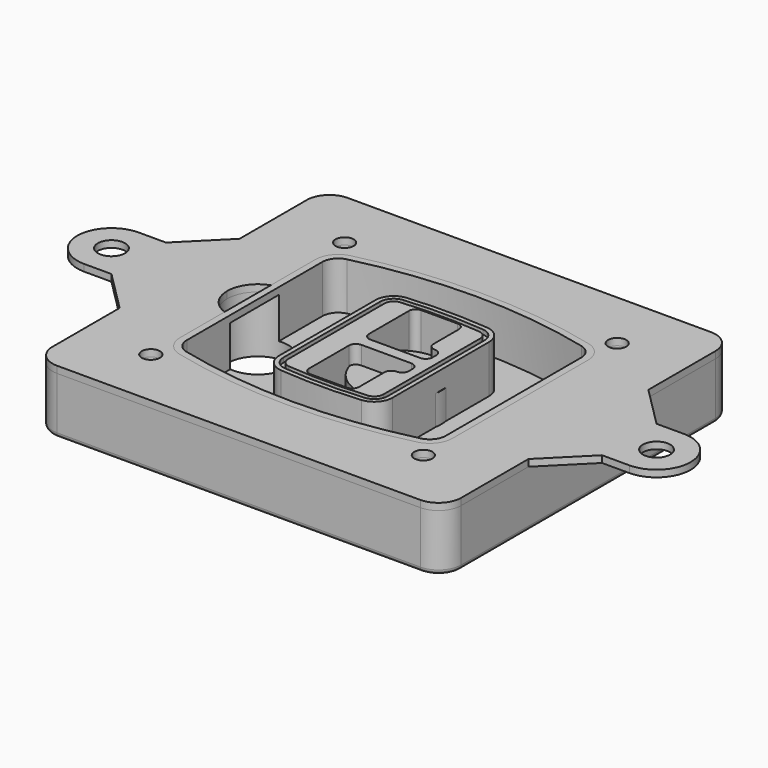
from build123d import *

# Parameters (mm, degrees)
F0_R      = 4
F1_DEPTH  = 25
F2_DEPTH  = 3
F3_DEPTH  = 18
F5_DEPTH  = 21
F6_DEPTH  = 2
F8_DEPTH  = 20
F9_DEPTH  = 16
F10_DEPTH = 25
F7_R      = 6
F7_R_2    = 4
F11_DEPTH = 6
F13_DEPTH = 9
F15_R     = 2
F16_R     = 4
F16_R_2   = 6
F17_DEPTH = 3


# Not quite as in the source:
# - a feature of the source that left no trace in its solid (it failed there, or was rolled back) is left out
# - a feature names something its author has since deleted; it is built from what else it names


with BuildPart() as f1:
    # F0 (on Top) → F1 (new body)
    with BuildSketch(Plane.XY):
        with BuildLine():
            ThreePointArc((-90, -70), (-87.0710678119, -77.0710678119), (-80, -80))
            Line((-80, -80), (80, -80))
            ThreePointArc((80, -80), (87.0710678119, -77.0710678119), (90, -70))
            Line((90, -70), (90, 70))
            ThreePointArc((90, 70), (87.0710678119, 77.0710678119), (80, 80))
            Line((80, 80), (-80, 80))
            ThreePointArc((-80, 80), (-87.0710678119, 77.0710678119), (-90, 70))
            Line((-90, 70), (-90, -70))
        make_face()
        with Locations((-60, -53.3333333333)):
            Circle(F0_R, mode=Mode.SUBTRACT)
        with Locations((60, -53.3333333333)):
            Circle(F0_R, mode=Mode.SUBTRACT)
        with Locations((-60, 53.3333333333)):
            Circle(F0_R, mode=Mode.SUBTRACT)
        with BuildLine():
            ThreePointArc((-64, 37.2990447398), (-61.0143011354, 45.9411029726), (-53.3306899286, 50.8970778549))
            ThreePointArc((-53.3306899286, 50.8970778549), (0, 57.3333333333), (53.3306899286, 50.8970778549))
            ThreePointArc((53.3306899286, 50.8970778549), (61.0143011354, 45.9411029726), (64, 37.2990447398))
            Line((64, 37.2990447398), (64, -37.2990447398))
            ThreePointArc((64, -37.2990447398), (61.0143011354, -45.9411029726), (53.3306899286, -50.8970778549))
            ThreePointArc((53.3306899286, -50.8970778549), (0, -57.3333333333), (-53.3306899286, -50.8970778549))
            ThreePointArc((-53.3306899286, -50.8970778549), (-61.0143011354, -45.9411029726), (-64, -37.2990447398))
            Line((-64, -37.2990447398), (-64, 37.2990447398))
        make_face(mode=Mode.SUBTRACT)
        with Locations((60, 53.3333333333)):
            Circle(F0_R, mode=Mode.SUBTRACT)
        with BuildLine():
            ThreePointArc((53.3306899286, 50.8970778549), (0, 57.3333333333), (-53.3306899286, 50.8970778549))
            ThreePointArc((-53.3306899286, 50.8970778549), (-61.0143011354, 45.9411029726), (-64, 37.2990447398))
            Line((-64, 37.2990447398), (-64, -37.2990447398))
            ThreePointArc((-64, -37.2990447398), (-61.0143011354, -45.9411029726), (-53.3306899286, -50.8970778549))
            ThreePointArc((-53.3306899286, -50.8970778549), (0, -57.3333333333), (53.3306899286, -50.8970778549))
            ThreePointArc((53.3306899286, -50.8970778549), (61.0143011354, -45.9411029726), (64, -37.2990447398))
            Line((64, -37.2990447398), (64, 37.2990447398))
            ThreePointArc((64, 37.2990447398), (61.0143011354, 45.9411029726), (53.3306899286, 50.8970778549))
        make_face()
        with BuildLine():
            Line((-60, -37.2990447398), (-60, 37.2990447398))
            ThreePointArc((-60, 37.2990447398), (-57.8673579538, 43.4719434775), (-52.3790642347, 47.0119255363))
            ThreePointArc((-52.3790642347, 47.0119255363), (0, 53.3333333333), (52.3790642347, 47.0119255363))
            ThreePointArc((52.3790642347, 47.0119255363), (57.8673579538, 43.4719434775), (60, 37.2990447398))
            Line((60, 37.2990447398), (60, -37.2990447398))
            ThreePointArc((60, -37.2990447398), (57.8673579538, -43.4719434775), (52.3790642347, -47.0119255363))
            ThreePointArc((52.3790642347, -47.0119255363), (0, -53.3333333333), (-52.3790642347, -47.0119255363))
            ThreePointArc((-52.3790642347, -47.0119255363), (-57.8673579538, -43.4719434775), (-60, -37.2990447398))
        make_face(mode=Mode.SUBTRACT)
        with BuildLine():
            ThreePointArc((-52.3790642347, 47.0119255363), (-57.8673579538, 43.4719434775), (-60, 37.2990447398))
            Line((-60, 37.2990447398), (-60, -37.2990447398))
            ThreePointArc((-60, -37.2990447398), (-57.8673579538, -43.4719434775), (-52.3790642347, -47.0119255363))
            ThreePointArc((-52.3790642347, -47.0119255363), (0, -53.3333333333), (52.3790642347, -47.0119255363))
            ThreePointArc((52.3790642347, -47.0119255363), (57.8673579538, -43.4719434775), (60, -37.2990447398))
            Line((60, -37.2990447398), (60, 37.2990447398))
            ThreePointArc((60, 37.2990447398), (57.8673579538, 43.4719434775), (52.3790642347, 47.0119255363))
            ThreePointArc((52.3790642347, 47.0119255363), (0, 53.3333333333), (-52.3790642347, 47.0119255363))
        make_face()
        with BuildLine():
            ThreePointArc((51.6653449643, 44.0980612973), (55.5071505677, 41.6200738562), (57, 37.2990447398))
            Line((57, 37.2990447398), (57, -37.2990447398))
            ThreePointArc((57, -37.2990447398), (55.5071505677, -41.6200738562), (51.6653449643, -44.0980612973))
            ThreePointArc((51.6653449643, -44.0980612973), (0, -50.3333333333), (-51.6653449643, -44.0980612973))
            ThreePointArc((-51.6653449643, -44.0980612973), (-55.5071505677, -41.6200738562), (-57, -37.2990447398))
            Line((-57, -37.2990447398), (-57, 37.2990447398))
            ThreePointArc((-57, 37.2990447398), (-55.5071505677, 41.6200738562), (-51.6653449643, 44.0980612973))
            ThreePointArc((-51.6653449643, 44.0980612973), (0, 50.3333333333), (51.6653449643, 44.0980612973))
        make_face(mode=Mode.SUBTRACT)
        with BuildLine():
            Line((57, -37.2990447398), (57, 37.2990447398))
            ThreePointArc((57, 37.2990447398), (55.5071505677, 41.6200738562), (51.6653449643, 44.0980612973))
            ThreePointArc((51.6653449643, 44.0980612973), (0, 50.3333333333), (-51.6653449643, 44.0980612973))
            ThreePointArc((-51.6653449643, 44.0980612973), (-55.5071505677, 41.6200738562), (-57, 37.2990447398))
            Line((-57, 37.2990447398), (-57, -37.2990447398))
            ThreePointArc((-57, -37.2990447398), (-55.5071505677, -41.6200738562), (-51.6653449643, -44.0980612973))
            ThreePointArc((-51.6653449643, -44.0980612973), (0, -50.3333333333), (51.6653449643, -44.0980612973))
            ThreePointArc((51.6653449643, -44.0980612973), (55.5071505677, -41.6200738562), (57, -37.2990447398))
        make_face()
    extrude(amount=-F1_DEPTH)

    # F0 (on Top) → F2 (join)
    with BuildSketch(Plane.XY):
        with BuildLine():
            ThreePointArc((-52.3790642347, 47.0119255363), (-57.8673579538, 43.4719434775), (-60, 37.2990447398))
            Line((-60, 37.2990447398), (-60, -37.2990447398))
            ThreePointArc((-60, -37.2990447398), (-57.8673579538, -43.4719434775), (-52.3790642347, -47.0119255363))
            ThreePointArc((-52.3790642347, -47.0119255363), (0, -53.3333333333), (52.3790642347, -47.0119255363))
            ThreePointArc((52.3790642347, -47.0119255363), (57.8673579538, -43.4719434775), (60, -37.2990447398))
            Line((60, -37.2990447398), (60, 37.2990447398))
            ThreePointArc((60, 37.2990447398), (57.8673579538, 43.4719434775), (52.3790642347, 47.0119255363))
            ThreePointArc((52.3790642347, 47.0119255363), (0, 53.3333333333), (-52.3790642347, 47.0119255363))
        make_face()
        with BuildLine():
            ThreePointArc((51.6653449643, 44.0980612973), (55.5071505677, 41.6200738562), (57, 37.2990447398))
            Line((57, 37.2990447398), (57, -37.2990447398))
            ThreePointArc((57, -37.2990447398), (55.5071505677, -41.6200738562), (51.6653449643, -44.0980612973))
            ThreePointArc((51.6653449643, -44.0980612973), (0, -50.3333333333), (-51.6653449643, -44.0980612973))
            ThreePointArc((-51.6653449643, -44.0980612973), (-55.5071505677, -41.6200738562), (-57, -37.2990447398))
            Line((-57, -37.2990447398), (-57, 37.2990447398))
            ThreePointArc((-57, 37.2990447398), (-55.5071505677, 41.6200738562), (-51.6653449643, 44.0980612973))
            ThreePointArc((-51.6653449643, 44.0980612973), (0, 50.3333333333), (51.6653449643, 44.0980612973))
        make_face(mode=Mode.SUBTRACT)
    extrude(amount=F2_DEPTH)

    # F0 (on Top) → F3 (cut)
    with BuildSketch(Plane.XY):
        with BuildLine():
            Line((57, -37.2990447398), (57, 37.2990447398))
            ThreePointArc((57, 37.2990447398), (55.5071505677, 41.6200738562), (51.6653449643, 44.0980612973))
            ThreePointArc((51.6653449643, 44.0980612973), (0, 50.3333333333), (-51.6653449643, 44.0980612973))
            ThreePointArc((-51.6653449643, 44.0980612973), (-55.5071505677, 41.6200738562), (-57, 37.2990447398))
            Line((-57, 37.2990447398), (-57, -37.2990447398))
            ThreePointArc((-57, -37.2990447398), (-55.5071505677, -41.6200738562), (-51.6653449643, -44.0980612973))
            ThreePointArc((-51.6653449643, -44.0980612973), (0, -50.3333333333), (51.6653449643, -44.0980612973))
            ThreePointArc((51.6653449643, -44.0980612973), (55.5071505677, -41.6200738562), (57, -37.2990447398))
        make_face()
    extrude(amount=-F3_DEPTH, mode=Mode.SUBTRACT)

    # F4 (on face) → F5 (join, through all)
    with BuildSketch(Plane.XY.offset(3)):
        with BuildLine():
            ThreePointArc((-25, -26.587695628), (-22.8992979869, -31.9912392117), (-17.7004291845, -34.5569740744))
            ThreePointArc((-17.7004291845, -34.5569740744), (0, -35.3333333333), (17.7004291845, -34.5569740744))
            ThreePointArc((17.7004291845, -34.5569740744), (22.8992979869, -31.9912392117), (25, -26.587695628))
            Line((25, -26.587695628), (25, 26.587695628))
            ThreePointArc((25, 26.587695628), (22.8992979869, 31.9912392117), (17.7004291845, 34.5569740744))
            ThreePointArc((17.7004291845, 34.5569740744), (0, 35.3333333333), (-17.7004291845, 34.5569740744))
            ThreePointArc((-17.7004291845, 34.5569740744), (-22.8992979869, 31.9912392117), (-25, 26.587695628))
            Line((-25, 26.587695628), (-25, -26.587695628))
        make_face()
        with BuildLine():
            ThreePointArc((17.5253218884, 32.5646544628), (21.4244734902, 30.6403533158), (23, 26.587695628))
            Line((23, 26.587695628), (23, -26.587695628))
            ThreePointArc((23, -26.587695628), (21.4244734902, -30.6403533158), (17.5253218884, -32.5646544628))
            ThreePointArc((17.5253218884, -32.5646544628), (0, -33.3333333333), (-17.5253218884, -32.5646544628))
            ThreePointArc((-17.5253218884, -32.5646544628), (-21.4244734902, -30.6403533158), (-23, -26.587695628))
            Line((-23, -26.587695628), (-23, 26.587695628))
            ThreePointArc((-23, 26.587695628), (-21.4244734902, 30.6403533158), (-17.5253218884, 32.5646544628))
            ThreePointArc((-17.5253218884, 32.5646544628), (0, 33.3333333333), (17.5253218884, 32.5646544628))
        make_face(mode=Mode.SUBTRACT)
        with BuildLine():
            Line((23, -26.587695628), (23, 26.587695628))
            ThreePointArc((23, 26.587695628), (21.4244734902, 30.6403533158), (17.5253218884, 32.5646544628))
            ThreePointArc((17.5253218884, 32.5646544628), (0, 33.3333333333), (-17.5253218884, 32.5646544628))
            ThreePointArc((-17.5253218884, 32.5646544628), (-21.4244734902, 30.6403533158), (-23, 26.587695628))
            Line((-23, 26.587695628), (-23, -26.587695628))
            ThreePointArc((-23, -26.587695628), (-21.4244734902, -30.6403533158), (-17.5253218884, -32.5646544628))
            ThreePointArc((-17.5253218884, -32.5646544628), (0, -33.3333333333), (17.5253218884, -32.5646544628))
            ThreePointArc((17.5253218884, -32.5646544628), (21.4244734902, -30.6403533158), (23, -26.587695628))
        make_face()
        with BuildLine():
            ThreePointArc((17.3502145923, 30.5723348512), (19.9496489934, 29.2894674198), (21, 26.587695628))
            Line((21, 26.587695628), (21, -26.587695628))
            ThreePointArc((21, -26.587695628), (19.9496489934, -29.2894674198), (17.3502145923, -30.5723348512))
            ThreePointArc((17.3502145923, -30.5723348512), (0, -31.3333333333), (-17.3502145923, -30.5723348512))
            ThreePointArc((-17.3502145923, -30.5723348512), (-19.9496489934, -29.2894674198), (-21, -26.587695628))
            Line((-21, -26.587695628), (-21, 26.587695628))
            ThreePointArc((-21, 26.587695628), (-19.9496489934, 29.2894674198), (-17.3502145923, 30.5723348512))
            ThreePointArc((-17.3502145923, 30.5723348512), (0, 31.3333333333), (17.3502145923, 30.5723348512))
        make_face(mode=Mode.SUBTRACT)
        with BuildLine():
            Line((21, -26.587695628), (21, 26.587695628))
            ThreePointArc((21, 26.587695628), (19.9496489934, 29.2894674198), (17.3502145923, 30.5723348512))
            ThreePointArc((17.3502145923, 30.5723348512), (0, 31.3333333333), (-17.3502145923, 30.5723348512))
            ThreePointArc((-17.3502145923, 30.5723348512), (-19.9496489934, 29.2894674198), (-21, 26.587695628))
            Line((-21, 26.587695628), (-21, -26.587695628))
            ThreePointArc((-21, -26.587695628), (-19.9496489934, -29.2894674198), (-17.3502145923, -30.5723348512))
            ThreePointArc((-17.3502145923, -30.5723348512), (0, -31.3333333333), (17.3502145923, -30.5723348512))
            ThreePointArc((17.3502145923, -30.5723348512), (19.9496489934, -29.2894674198), (21, -26.587695628))
        make_face()
        with BuildLine():
            Line((-8, -2.5), (14, -2.5))
            ThreePointArc((14, -2.5), (16.1213203436, -3.3786796564), (17, -5.5))
            Line((17, -5.5), (17, -7.5))
            ThreePointArc((17, -7.5), (16.1213203436, -9.6213203436), (14, -10.5))
            ThreePointArc((14, -10.5), (11.8786796564, -11.3786796564), (11, -13.5))
            Line((11, -13.5), (11, -27.5))
            ThreePointArc((11, -27.5), (10.1213203436, -29.6213203436), (8, -30.5))
            Line((8, -30.5), (-8, -30.5))
            ThreePointArc((-8, -30.5), (-10.1213203436, -29.6213203436), (-11, -27.5))
            Line((-11, -27.5), (-11, -5.5))
            ThreePointArc((-11, -5.5), (-10.1213203436, -3.3786796564), (-8, -2.5))
        make_face(mode=Mode.SUBTRACT)
        with BuildLine():
            ThreePointArc((-8, 2.5), (-10.1213203436, 3.3786796564), (-11, 5.5))
            Line((-11, 5.5), (-11, 27.5))
            ThreePointArc((-11, 27.5), (-10.1213203436, 29.6213203436), (-8, 30.5))
            Line((-8, 30.5), (8, 30.5))
            ThreePointArc((8, 30.5), (10.1213203436, 29.6213203436), (11, 27.5))
            Line((11, 27.5), (11, 13.5))
            ThreePointArc((11, 13.5), (11.8786796564, 11.3786796564), (14, 10.5))
            ThreePointArc((14, 10.5), (16.1213203436, 9.6213203436), (17, 7.5))
            Line((17, 7.5), (17, 5.5))
            ThreePointArc((17, 5.5), (16.1213203436, 3.3786796564), (14, 2.5))
            Line((14, 2.5), (-8, 2.5))
        make_face(mode=Mode.SUBTRACT)
    extrude(amount=-F5_DEPTH)

    # F4 (on face) → F6 (cut)
    with BuildSketch(Plane.XY.offset(3)):
        with BuildLine():
            Line((23, -26.587695628), (23, 26.587695628))
            ThreePointArc((23, 26.587695628), (21.4244734902, 30.6403533158), (17.5253218884, 32.5646544628))
            ThreePointArc((17.5253218884, 32.5646544628), (0, 33.3333333333), (-17.5253218884, 32.5646544628))
            ThreePointArc((-17.5253218884, 32.5646544628), (-21.4244734902, 30.6403533158), (-23, 26.587695628))
            Line((-23, 26.587695628), (-23, -26.587695628))
            ThreePointArc((-23, -26.587695628), (-21.4244734902, -30.6403533158), (-17.5253218884, -32.5646544628))
            ThreePointArc((-17.5253218884, -32.5646544628), (0, -33.3333333333), (17.5253218884, -32.5646544628))
            ThreePointArc((17.5253218884, -32.5646544628), (21.4244734902, -30.6403533158), (23, -26.587695628))
        make_face()
        with BuildLine():
            ThreePointArc((17.3502145923, 30.5723348512), (19.9496489934, 29.2894674198), (21, 26.587695628))
            Line((21, 26.587695628), (21, -26.587695628))
            ThreePointArc((21, -26.587695628), (19.9496489934, -29.2894674198), (17.3502145923, -30.5723348512))
            ThreePointArc((17.3502145923, -30.5723348512), (0, -31.3333333333), (-17.3502145923, -30.5723348512))
            ThreePointArc((-17.3502145923, -30.5723348512), (-19.9496489934, -29.2894674198), (-21, -26.587695628))
            Line((-21, -26.587695628), (-21, 26.587695628))
            ThreePointArc((-21, 26.587695628), (-19.9496489934, 29.2894674198), (-17.3502145923, 30.5723348512))
            ThreePointArc((-17.3502145923, 30.5723348512), (0, 31.3333333333), (17.3502145923, 30.5723348512))
        make_face(mode=Mode.SUBTRACT)
    extrude(amount=-F6_DEPTH, mode=Mode.SUBTRACT)

    # F7 (on face) → F8 (join)
    with BuildSketch(Plane(origin=(0, 0, -25), x_dir=(1, 0, 0), z_dir=(0, 0, -1))):
        with BuildLine():
            ThreePointArc((-6.71157564, 0), (6.7567035675, 13.4682792075), (20.224982775, 0))
            Line((20.224982775, 0), (25.224982775, 0))
            ThreePointArc((25.224982775, 0), (6.7567035675, 18.4682792075), (-11.71157564, 0))
            Line((-11.71157564, 0), (-6.71157564, 0))
        make_face()
        with BuildLine():
            Line((-6.71157564, 0), (20.224982775, 0))
            ThreePointArc((20.224982775, 0), (6.7567035675, 13.4682792075), (-6.71157564, 0))
        make_face()
        with BuildLine():
            ThreePointArc((-6.71157564, 0), (6.7567035675, -13.4682792075), (20.224982775, 0))
            Line((20.224982775, 0), (-6.71157564, 0))
        make_face()
        with BuildLine():
            Line((25.224982775, 0), (20.224982775, 0))
            ThreePointArc((20.224982775, 0), (6.7567035675, -13.4682792075), (-6.71157564, 0))
            Line((-6.71157564, 0), (-11.71157564, 0))
            ThreePointArc((-11.71157564, 0), (6.7567035675, -18.4682792075), (25.224982775, 0))
        make_face()
    extrude(amount=-F8_DEPTH)

    # F7 (on face) → F9 (cut)
    with BuildSketch(Plane(origin=(0, 0, -25), x_dir=(1, 0, 0), z_dir=(0, 0, -1))):
        with BuildLine():
            Line((-6.71157564, 0), (20.224982775, 0))
            ThreePointArc((20.224982775, 0), (6.7567035675, 13.4682792075), (-6.71157564, 0))
        make_face()
        with BuildLine():
            ThreePointArc((-6.71157564, 0), (6.7567035675, -13.4682792075), (20.224982775, 0))
            Line((20.224982775, 0), (-6.71157564, 0))
        make_face()
    extrude(amount=-F9_DEPTH, mode=Mode.SUBTRACT)

    # F7 (on face) → F10 (cut)
    with BuildSketch(Plane(origin=(0, 0, -25), x_dir=(1, 0, 0), z_dir=(0, 0, -1))):
        with BuildLine():
            Line((-69.0318229325, 0), (-42.0952645175, 0))
            ThreePointArc((-42.0952645175, 0), (-55.563543725, 13.4682792075), (-69.0318229325, 0))
        make_face()
        with BuildLine():
            ThreePointArc((-69.0318229325, 0), (-55.563543725, -13.4682792075), (-42.0952645175, 0))
            Line((-42.0952645175, 0), (-69.0318229325, 0))
        make_face()
    extrude(amount=-F10_DEPTH, mode=Mode.SUBTRACT)

    # F7 (on face) → F11 (cut)
    with BuildSketch(Plane(origin=(0, 0, -25), x_dir=(1, 0, 0), z_dir=(0, 0, -1))):
        with Locations((60, -53.3333333333)):
            Circle(F7_R)
        with Locations((60, -53.3333333333)):
            Circle(F7_R_2, mode=Mode.SUBTRACT)
        with Locations((-60, -53.3333333333)):
            Circle(F7_R)
        with Locations((-60, -53.3333333333)):
            Circle(F7_R_2, mode=Mode.SUBTRACT)
        with Locations((-60, 53.3333333333)):
            Circle(F7_R)
        with Locations((-60, 53.3333333333)):
            Circle(F7_R_2, mode=Mode.SUBTRACT)
        with Locations((60, 53.3333333333)):
            Circle(F7_R)
        with Locations((60, 53.3333333333)):
            Circle(F7_R_2, mode=Mode.SUBTRACT)
    extrude(amount=-F11_DEPTH, mode=Mode.SUBTRACT)

    # F12 (on face) → F13 (cut, through all)
    with BuildSketch(Plane(origin=(0, 0, -9), x_dir=(1, 0, 0), z_dir=(0, 0, -1))):
        with BuildLine():
            ThreePointArc((20.224982775, 0), (20.1663399806, 1.2554664788), (19.9909222755, 2.5))
            Line((19.9909222755, 2.5), (14, 2.5))
            ThreePointArc((14, 2.5), (16.1213203436, 3.3786796564), (17, 5.5))
            Line((17, 5.5), (17, 7.5))
            ThreePointArc((17, 7.5), (16.1213203436, 9.6213203436), (14, 10.5))
            ThreePointArc((14, 10.5), (12.1627255951, 11.1284134507), (11.0951631559, 12.750384826))
            ThreePointArc((11.0951631559, 12.750384826), (11.0476113807, 12.7664660322), (11, 12.7823698976))
            Line((11, 12.7823698976), (11, -12.7823698976))
            ThreePointArc((11, -12.7823698976), (11.0476113807, -12.7664660322), (11.0951631559, -12.750384826))
            ThreePointArc((11.0951631559, -12.750384826), (12.1627255951, -11.1284134507), (14, -10.5))
            ThreePointArc((14, -10.5), (16.1213203436, -9.6213203436), (17, -7.5))
            Line((17, -7.5), (17, -5.5))
            ThreePointArc((17, -5.5), (16.1213203436, -3.3786796564), (14, -2.5))
            Line((14, -2.5), (19.9909222755, -2.5))
            ThreePointArc((19.9909222755, -2.5), (20.1663399806, -1.2554664788), (20.224982775, 0))
        make_face()
    extrude(amount=F13_DEPTH, mode=Mode.SUBTRACT)

    # F15
    f15_edges = [f1.edges().sort_by_distance(p)[0] for p in [
        (0, -80, -25),
        (-87.071068, -77.071068, -25),
        (-90, 0, -25),
        (-87.071068, 77.071068, -25),
        (87.071068, -77.071068, -25),
        (0, 80, -25),
        (90, 0, -25),
        (87.071068, 77.071068, -25),
    ]]
    fillet(f15_edges, radius=F15_R)


with BuildPart() as f17:
    # F16 (on face) → F17 (new body, through all)
    with BuildSketch(Plane.XY):
        with BuildLine():
            Line((90, -33), (90, 33))
            Line((90, 33), (90, 70))
            ThreePointArc((90, 70), (87.0710678119, 77.0710678119), (80, 80))
            Line((80, 80), (-80, 80))
            ThreePointArc((-80, 80), (-87.0710678119, 77.0710678119), (-90, 70))
            Line((-90, 70), (-90, 33))
            Line((-90, 33), (-90, -33))
            Line((-90, -33), (-90, -70))
            ThreePointArc((-90, -70), (-87.0710678119, -77.0710678119), (-80, -80))
            Line((-80, -80), (80, -80))
            ThreePointArc((80, -80), (87.0710678119, -77.0710678119), (90, -70))
            Line((90, -70), (90, -33))
        make_face()
        with Locations((-60, -53.3333333333)):
            Circle(F16_R, mode=Mode.SUBTRACT)
        with BuildLine():
            ThreePointArc((-60, 37.2990447398), (-57.8673579538, 43.4719434775), (-52.3790642347, 47.0119255363))
            ThreePointArc((-52.3790642347, 47.0119255363), (0, 53.3333333333), (52.3790642347, 47.0119255363))
            ThreePointArc((52.3790642347, 47.0119255363), (57.8673579538, 43.4719434775), (60, 37.2990447398))
            Line((60, 37.2990447398), (60, -37.2990447398))
            ThreePointArc((60, -37.2990447398), (57.8673579538, -43.4719434775), (52.3790642347, -47.0119255363))
            ThreePointArc((52.3790642347, -47.0119255363), (0, -53.3333333333), (-52.3790642347, -47.0119255363))
            ThreePointArc((-52.3790642347, -47.0119255363), (-57.8673579538, -43.4719434775), (-60, -37.2990447398))
            Line((-60, -37.2990447398), (-60, -12.7166190685))
            ThreePointArc((-60, -12.7166190685), (-66.5441169481, -7.798817635), (-69.0318229325, 0))
            ThreePointArc((-69.0318229325, 0), (-66.5441169481, 7.798817635), (-60, 12.7166190685))
            Line((-60, 12.7166190685), (-60, 37.2990447398))
        make_face(mode=Mode.SUBTRACT)
        with Locations((60, -53.3333333333)):
            Circle(F16_R, mode=Mode.SUBTRACT)
        with Locations((-60, 53.3333333333)):
            Circle(F16_R, mode=Mode.SUBTRACT)
        with Locations((60, 53.3333333333)):
            Circle(F16_R, mode=Mode.SUBTRACT)
        with BuildLine():
            Line((-90, -33), (-90, 33))
            Line((-90, 33), (-108, 15))
            Line((-108, 15), (-120, 15))
            ThreePointArc((-120, 15), (-135, 0), (-120, -15))
            Line((-120, -15), (-108, -15))
            Line((-108, -15), (-90, -33))
        make_face()
        with Locations((-120, 0)):
            Circle(F16_R_2, mode=Mode.SUBTRACT)
        with BuildLine():
            Line((108, 15), (90, 33))
            Line((90, 33), (90, -33))
            Line((90, -33), (108, -15))
            Line((108, -15), (120, -15))
            ThreePointArc((120, -15), (135, 0), (120, 15))
            Line((120, 15), (108, 15))
        make_face()
        with Locations((120, 0)):
            Circle(F16_R_2, mode=Mode.SUBTRACT)
    extrude(amount=F17_DEPTH)


solid = Compound([f1.part, f17.part])
